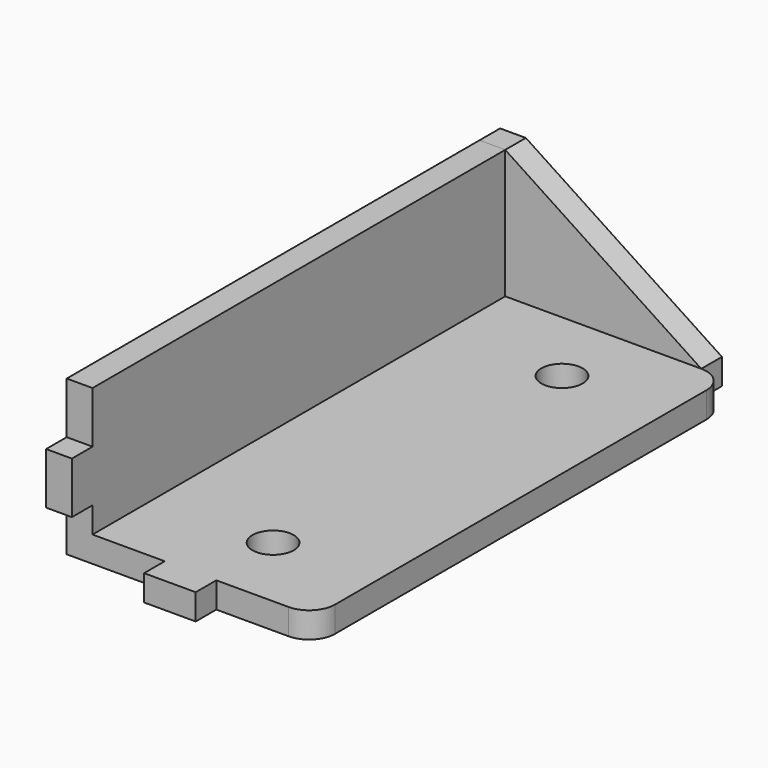
from build123d import *

# Parameters (mm, degrees)
F1_DEPTH = 100
F2_R     = 4
F3_DEPTH = 25
F4_R     = 5
F6_DEPTH = 5
F8_W     = 5
F8_H     = 10
F8_W_2   = 14
F8_H_2   = 5
F9_DEPTH = 5


# Not quite as in the source:
# - a pattern or mirror of a feature is missing from the dataset's text; its kind, count and spacing are read off the source's solid


with BuildPart() as f1:
    # F0 (on Front) → F1 (new body)
    with BuildSketch(Plane.XZ):
        Polygon((0, 30), (0, 0), (48, 0), (48, 5), (5, 5), (5, 30), align=None)
    extrude(amount=F1_DEPTH)

    # F2 (on face) → F3 (cut)
    with BuildSketch(Plane.XY.offset(5)):
        with Locations((28, -85)):
            Circle(F2_R)
        with Locations((28, -15)):
            Circle(F2_R)
    extrude(amount=-F3_DEPTH, mode=Mode.SUBTRACT)

    # F4
    f4_edges = [f1.edges().sort_by_distance(p)[0] for p in [
        (48, -100, 2.5),
        (48, 0, 2.5),
    ]]
    fillet(f4_edges, radius=F4_R)

    # F5 (on face) → F6 (join)
    with BuildSketch(Plane(origin=(0, 0, 0), x_dir=(-1, 0, 0), z_dir=(0, 1, 0))):
        Polygon((0, 10), (0, 15), (0, 20), (-5, 20), (-5, 10), align=None)
        Polygon((-19, 5), (-24, 5), (-29, 5), (-29, 0), (-19, 0), align=None)
    f6 = extrude(amount=F6_DEPTH)

    # F6_copies: F6 across plane
    add(f6.mirror(Plane(origin=(0, -50, 0), x_dir=(0, 0, -1), z_dir=(0, -1, 0))))


with BuildPart() as f9:
    # F8 (on face) → F9 (new body)
    with BuildSketch(Plane(origin=(0, 0, 0), x_dir=(-1, 0, 0), z_dir=(0, 1, 0))):
        Polygon((-5, 20), (-5, 30), (-43, 5), (-29, 5), (-19, 5), (-5, 5), (-5, 10), align=None)
        with Locations((-2.5, 25)):
            Rectangle(F8_W, F8_H)
        Polygon((0, 10), (-5, 10), (-5, 5), (-19, 5), (-19, 0), (0, 0), align=None)
        with Locations((-36, 2.5)):
            Rectangle(F8_W_2, F8_H_2)
    extrude(amount=F9_DEPTH)


solid = Compound([f1.part, f9.part])
